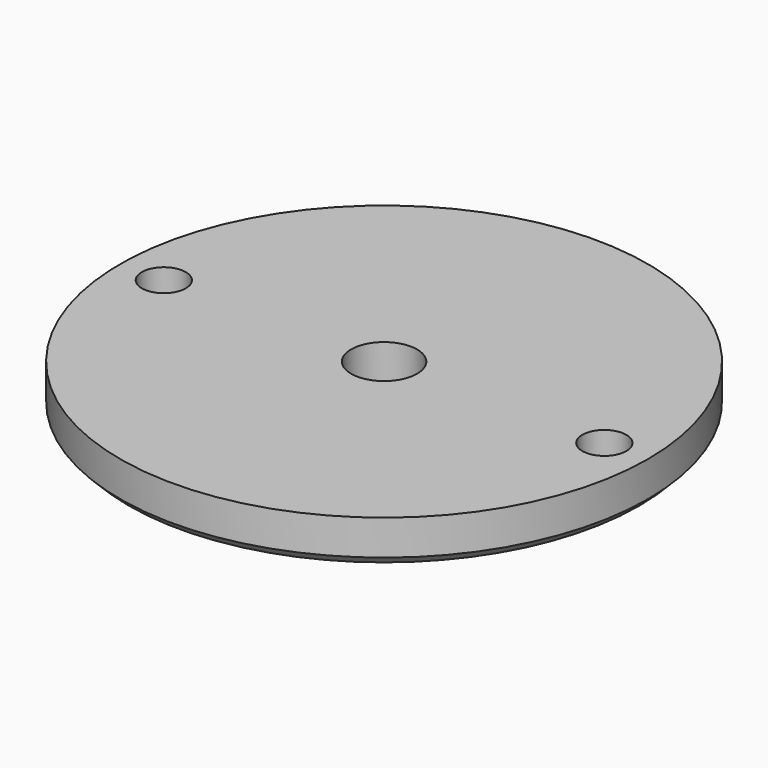
from build123d import *

# Parameters (mm, degrees)
F0_R     = 38.1
F1_DEPTH = 6.35
F2_R     = 3.175
F2_R_2   = 4.7625
F3_DEPTH = 25.4
F4_SIZE  = 1.27


# Not quite as in the source:
# - a length typed as a fraction of an inch, garbled in the dataset ("3 / 203.2 mm" for 3/8 in), is restored


with BuildPart() as f1:
    # F0 (on Top) → F1 (new body)
    with BuildSketch(Plane.XY):
        Circle(F0_R)
    extrude(amount=F1_DEPTH)

    # F2 (on Top) → F3 (cut)
    with BuildSketch(Plane.XY):
        with Locations((-31.7926891148, 0)):
            Circle(F2_R)
        with Locations((31.7926891148, 0)):
            Circle(F2_R)
        Circle(F2_R_2)
    extrude(amount=F3_DEPTH, mode=Mode.SUBTRACT)

    # F4
    f4_edges = [f1.edges().sort_by_distance(p)[0] for p in [
        (-38.1, 0, 0),
    ]]
    chamfer(f4_edges, length=F4_SIZE)


solid = f1.part
